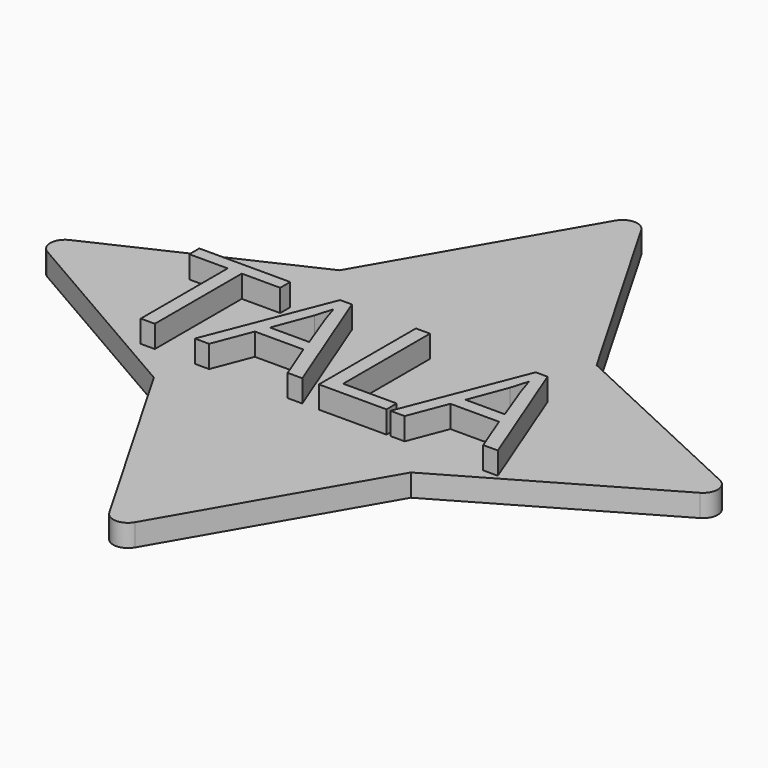
from build123d import *

# Parameters (mm, degrees)
F1_DEPTH     = 3
F2_TEXT_SIZE = 22.8898426323
F3_DEPTH     = 3


# Not quite as in the source:
# - Text() gives the source's letters only with a copy of the font that has no kerning and outlines rounded to 1/6400 em; it was checked with that copy


with BuildPart() as f1:
    # F0 (on Top) → F1 (new body)
    with BuildSketch(Plane.XY):
        with BuildLine():
            Line((15.5884572681, 27), (0, 0))
            Line((0, 0), (-26.5179978791, -12.36554549))
            ThreePointArc((-26.5179978791, -12.36554549), (-27.6708577988, -14.0909222893), (-26.6727613557, -15.9102118716))
            Line((-26.6727613557, -15.9102118716), (0, -31.3097378203))
            Line((0, -31.3097378203), (15.5884572681, -58.3097378203))
            ThreePointArc((15.5884572681, -58.3097378203), (17.3205080757, -59.3097378203), (19.0525588833, -58.3097378203))
            Line((19.0525588833, -58.3097378203), (34.6410161514, -31.3097378203))
            Line((34.6410161514, -31.3097378203), (61.313777507, -15.9102118716))
            ThreePointArc((61.313777507, -15.9102118716), (62.3118739502, -14.0909222893), (61.1590140305, -12.36554549))
            Line((61.1590140305, -12.36554549), (34.6410161514, 0))
            Line((34.6410161514, 0), (19.0525588833, 27))
            ThreePointArc((19.0525588833, 27), (17.3205080757, 28), (15.5884572681, 27))
        make_face()
    extrude(amount=F1_DEPTH)

    # F2 (on face) → F3 (join)
    with BuildSketch(Plane.XY.offset(3)):
        with Locations((-11.2484150256, -26.1787499559)):
            Text('TALA', F2_TEXT_SIZE, font='Open Sans', text_align=(TextAlign.LEFT, TextAlign.BOTTOM))
    extrude(amount=F3_DEPTH)


solid = f1.part
